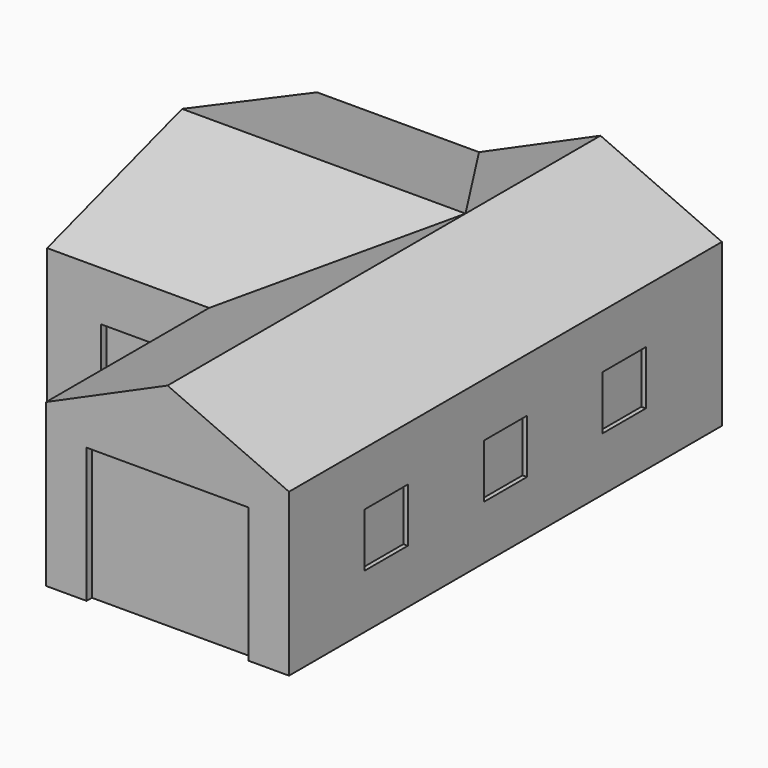
from build123d import *

# Parameters (mm, degrees)
F1_DEPTH      = 12192
F3_DEPTH      = 3657.6
F3_DEPTH_BACK = 2743.2
F4_DEPTH      = 30.48
F5_W          = 3657.6
F5_H          = 3048
F6_DEPTH      = 152.4
F7_W          = 3048
F7_H          = 3048
F8_DEPTH      = 152.4
F9_W          = 1219.2
F9_H          = 2438.4
F10_DEPTH     = 152.4
F11_W         = 1219.2
F11_H         = 1219.2
F12_DEPTH     = 100.584
F13_W         = 1219.2
F13_H         = 1219.2
F14_DEPTH     = 100.584
F15_W         = 1219.2
F15_H         = 1219.2
F16_DEPTH     = 100.584


with BuildPart() as f1:
    # F0 (on Front) → F1 (new body)
    with BuildSketch(Plane.XZ):
        Polygon((0, 3657.6), (0, 0), (5486.4, 0), (5486.4, 3657.6), (2743.2, 4876.8), align=None)
    extrude(amount=F1_DEPTH)

    # F2 (on face) → F3 (join, two sides)
    with BuildSketch(Plane(origin=(0, 0, 0), x_dir=(0, -1, 0), z_dir=(-1, 0, 0))) as f3_sk:
        Polygon((0, 3657.6), (0, 0), (7620, 0), (7620, 3657.6), (3810, 4876.8), align=None)
    extrude(amount=F3_DEPTH)
    extrude(f3_sk.sketch, amount=-F3_DEPTH_BACK)

    # F4 (add): a face of the model
    f4_faces = [f1.faces().sort_by_distance(p)[0] for p in [
        (2743.2, -12192, 2148.1142857143),
    ]]
    extrude(f4_faces, amount=F4_DEPTH)

    # F5 (on face) → F6 (cut)
    with BuildSketch(Plane.XZ.offset(12222.48)):
        with Locations((2743.2, 1524)):
            Rectangle(F5_W, F5_H)
    extrude(amount=-F6_DEPTH, mode=Mode.SUBTRACT)

    # F7 (on face) → F8 (cut)
    with BuildSketch(Plane(origin=(-3657.6, 0, 0), x_dir=(0, -1, 0), z_dir=(-1, 0, 0))):
        with Locations((3810, 1524)):
            Rectangle(F7_W, F7_H)
    extrude(amount=-F8_DEPTH, mode=Mode.SUBTRACT)

    # F9 (on face) → F10 (cut)
    with BuildSketch(Plane.XZ.offset(7620)):
        with Locations((-1828.8, 1319.784)):
            Rectangle(F9_W, F9_H)
    extrude(amount=-F10_DEPTH, mode=Mode.SUBTRACT)

    # F11 (on face) → F12 (cut)
    with BuildSketch(Plane.YZ.offset(5486.4)):
        with Locations((-9479.28, 1828.8)):
            Rectangle(F11_W, F11_H)
        with Locations((-6111.24, 1828.8)):
            Rectangle(F11_W, F11_H)
        with Locations((-2758.44, 1828.8)):
            Rectangle(F11_W, F11_H)
    extrude(amount=-F12_DEPTH, mode=Mode.SUBTRACT)

    # F13 (on face) → F14 (cut)
    with BuildSketch(Plane(origin=(0, 0, 0), x_dir=(-1, 0, 0), z_dir=(0, 1, 0))):
        with Locations((-2743.2, 1828.8)):
            Rectangle(F13_W, F13_H)
        with Locations((1524, 1828.8)):
            Rectangle(F13_W, F13_H)
    extrude(amount=-F14_DEPTH, mode=Mode.SUBTRACT)

    # F15 (on face) → F16 (cut)
    with BuildSketch(Plane(origin=(0, 0, 0), x_dir=(0, -1, 0), z_dir=(-1, 0, 0))):
        with Locations((9936.48, 1828.8)):
            Rectangle(F15_W, F15_H)
    extrude(amount=-F16_DEPTH, mode=Mode.SUBTRACT)


solid = f1.part
